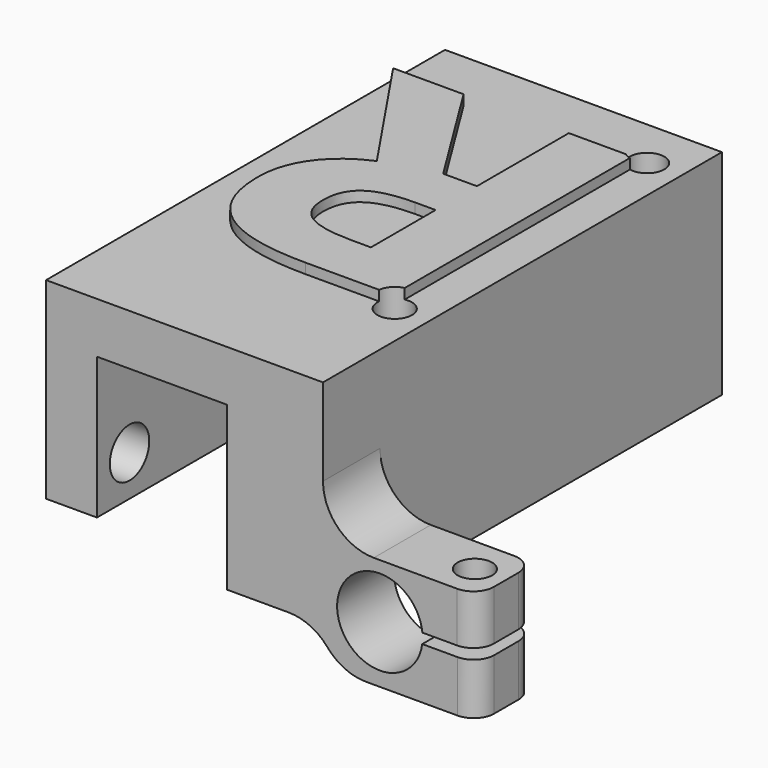
from build123d import *

# Parameters (mm, degrees)
F1_DEPTH      = 7
F2_DEPTH      = 42
F3_R          = 1.7
F3_R_2        = 11
F4_DEPTH      = 21.001
F5_R          = 4.2
F6_DEPTH      = 10
F7_DEPTH      = 21.001
F8_R          = 1.4
F9_DEPTH      = 11.0232760457
F8_R_2        = 1.7
F10_DEPTH     = 4.91123055
F11_R         = 5
F12_R         = 5
F13_R         = 5
F14_R         = 2
F15_R         = 2.2
F15_R_2       = 2.4255023423
F16_DEPTH     = 6
F17_TEXT_SIZE = 41.2177505736
F18_DEPTH     = 1
F19_DEPTH     = 22.0010001


# Not quite as in the source:
# - a feature names something its author has since deleted; it is built from what else it names
# - Text() gives the source's letters only with a copy of the font that has no kerning and outlines rounded to 1/6400 em; it was checked with that copy


with BuildPart() as f1:
    # F0 (on Front) → F1 (new body)
    with BuildSketch(Plane.XZ):
        Polygon((-18.6721007523, 29.8099789735), (-18.6721007523, 10.8925135386), (-13.6721007523, 10.8925135386), (-13.6721007523, 24.8099789735), (-0.8721007523, 24.8099789735), (-0.8721007523, 8.8099789735), (8.5380548998, 8.8099789735), (8.5380548998, 16.2656020473), (8.5380548998, 29.8099789735), align=None)
        Polygon((23.7263195603, 16.2417280634), (8.5380548998, 16.2656020473), (8.5380548998, 8.8099789735), (9.9533044869, 5.2860832236), (23.7553367778, 5.2860832236), (23.7553367778, 10.343908232), (17.0860510706, 10.343908232), (17.0860510706, 11.3388913612), (23.7263195603, 11.3388913612), align=None)
    extrude(amount=F1_DEPTH)

    # F0 (on Front) → F2 (join)
    with BuildSketch(Plane.XZ):
        Polygon((-18.6721007523, 29.8099789735), (-18.6721007523, 10.8925135386), (-13.6721007523, 10.8925135386), (-13.6721007523, 24.8099789735), (-0.8721007523, 24.8099789735), (-0.8721007523, 8.8099789735), (8.5380548998, 8.8099789735), (8.5380548998, 16.2656020473), (8.5380548998, 29.8099789735), align=None)
    extrude(amount=-F2_DEPTH)

    # F3 (on face) → F4 (cut, through all)
    with BuildSketch(Plane(origin=(0, 0, 8.8099789735), x_dir=(1, 0, 0), z_dir=(0, 0, -1))):
        with Locations((5.1850692477, -6)):
            Circle(F3_R)
        with Locations((5.1850692477, -37)):
            Circle(F3_R)
        with Locations((20.6850692477, -21.5)):
            Circle(F3_R_2)
    extrude(amount=-F4_DEPTH, mode=Mode.SUBTRACT)

    # F5 (on face) → F6 (cut)
    with BuildSketch(Plane.XZ.offset(7)):
        with Locations((14.1278992477, 10.8989789735)):
            Circle(F5_R)
    extrude(amount=-F6_DEPTH, mode=Mode.SUBTRACT)

    # F3 (on face) → F7 (cut, through all)
    with BuildSketch(Plane(origin=(0, 0, 8.8099789735), x_dir=(1, 0, 0), z_dir=(0, 0, -1))):
        with Locations((5.1850692477, -6)):
            Circle(F3_R)
        with Locations((5.1850692477, -37)):
            Circle(F3_R)
        with Locations((20.6850692477, -21.5)):
            Circle(F3_R_2)
    extrude(amount=-F7_DEPTH, mode=Mode.SUBTRACT)

    # F8 (on face) → F9 (cut, through all)
    with BuildSketch(Plane(origin=(0.0255884511, 0, 16.2789825415), x_dir=(0.9999987646, 0, -0.0015718685), z_dir=(0.0015718685, 0, 0.9999987646))):
        with Locations((20.7007603888, -3.5767070949)):
            Circle(F8_R)
    extrude(amount=-F9_DEPTH, mode=Mode.SUBTRACT)

    # F8 (on face) → F10 (cut, through all)
    with BuildSketch(Plane(origin=(0.0255884511, 0, 16.2789825415), x_dir=(0.9999987646, 0, -0.0015718685), z_dir=(0.0015718685, 0, 0.9999987646))):
        with Locations((20.7007603888, -3.5767070949)):
            Circle(F8_R_2)
        with Locations((20.7007603888, -3.5767070949)):
            Circle(F8_R, mode=Mode.SUBTRACT)
    extrude(amount=-F10_DEPTH, mode=Mode.SUBTRACT)

    # F11
    f11_edges = [f1.edges().sort_by_distance(p)[0] for p in [
        (8.538055, -3.5, 16.265602),
    ]]
    fillet(f11_edges, radius=F11_R)

    # F12
    f12_edges = [f1.edges().sort_by_distance(p)[0] for p in [
        (8.538055, -3.5, 8.809979),
    ]]
    fillet(f12_edges, radius=F12_R)

    # F13
    f13_edges = [f1.edges().sort_by_distance(p)[0] for p in [
        (9.953304, -3.5, 5.286083),
    ]]
    fillet(f13_edges, radius=F13_R)

    # F14
    f14_edges = [f1.edges().sort_by_distance(p)[0] for p in [
        (23.72632, -7, 13.79031),
        (23.755337, -7, 7.814996),
        (23.72632, 0, 13.79031),
        (23.755337, 0, 7.814996),
    ]]
    fillet(f14_edges, radius=F14_R)

    # F15 (on face) → F16 (cut)
    with BuildSketch(Plane(origin=(-18.6721007523, 0, 0), x_dir=(0, -1, 0), z_dir=(-1, 0, 0))):
        with Locations((-38, 14.8925135386)):
            Circle(F15_R)
        with Locations((3, 14.8925135386)):
            Circle(F15_R_2)
    extrude(amount=-F16_DEPTH, mode=Mode.SUBTRACT)

    # F17 (on face) → F18 (join)
    with BuildSketch(Plane.XY.offset(29.8099789735)):
        with Locations(Location((8.5380548998, 35.6269137775), (0, 0, 180))):
            Text('R', F17_TEXT_SIZE, font='Open Sans', font_style=FontStyle.BOLD, text_align=(TextAlign.LEFT, TextAlign.BOTTOM))
    extrude(amount=F18_DEPTH)

    # F3 (on face) → F19 (cut, through all)
    with BuildSketch(Plane(origin=(0, 0, 8.8099789735), x_dir=(1, 0, 0), z_dir=(0, 0, -1))):
        with Locations((5.1850692477, -6)):
            Circle(F3_R)
        with Locations((5.1850692477, -37)):
            Circle(F3_R)
        with Locations((20.6850692477, -21.5)):
            Circle(F3_R_2)
    extrude(amount=-F19_DEPTH, mode=Mode.SUBTRACT)


solid = f1.part
